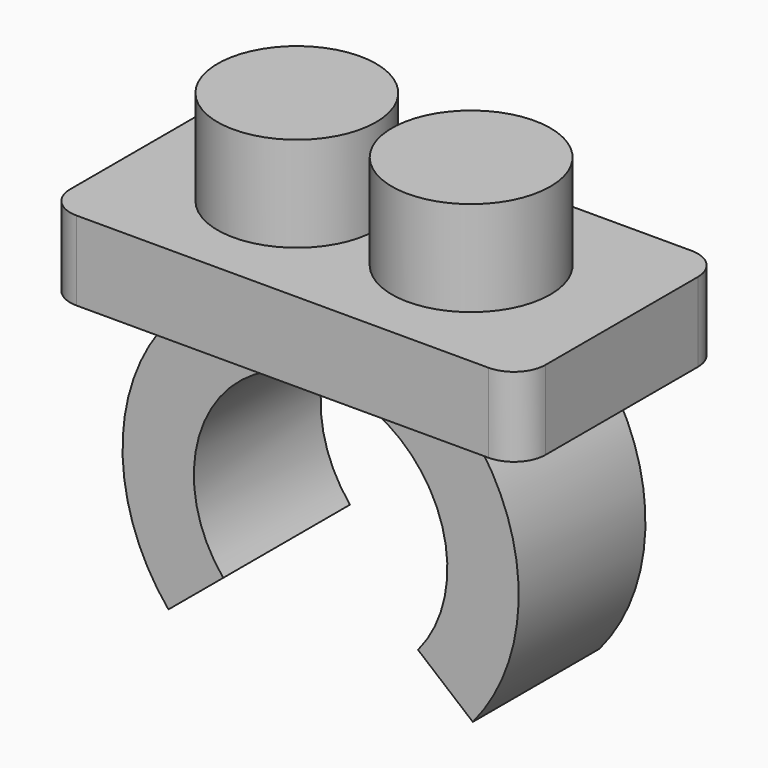
from build123d import *

# Parameters (mm, degrees)
F0_R     = 2.5
F1_DEPTH = 3
F2_W     = 15
F2_H     = 8
F3_DEPTH = 2.5
F5_DEPTH = 2.5
F6_R     = 1


with BuildPart() as f1:
    # F0 (on Top) → F1 (new body, symmetric)
    with BuildSketch(Plane.XY):
        with Locations((-2.75, 0)):
            Circle(F0_R)
    extrude(amount=F1_DEPTH, both=True)


with BuildPart() as f1b:
    # F0 (on Top) → F1, piece 2 (new body, symmetric)
    with BuildSketch(Plane.XY):
        with Locations((2.75, 0)):
            Circle(F0_R)
    extrude(amount=F1_DEPTH, both=True)


with BuildPart() as f3:
    # F2 (on Top) → F3 (new body)
    with BuildSketch(Plane.XY):
        Rectangle(F2_W, F2_H)
    extrude(amount=-F3_DEPTH)

    # F4 (on Front) → F5 (join, symmetric)
    with BuildSketch(Plane.XZ):
        with BuildLine():
            ThreePointArc((-3.073499634, -9.56), (0, -3), (3.073499634, -9.56))
            Line((3.073499634, -9.56), (4.8023431781, -11))
            ThreePointArc((4.8023431781, -11), (0, -0.75), (-4.8023431781, -11))
            Line((-4.8023431781, -11), (-3.073499634, -9.56))
        make_face()
    extrude(amount=F5_DEPTH, both=True)

    # F6
    f6_edges = [f3.edges().sort_by_distance(p)[0] for p in [
        (7.5, -4, -1.25),
        (-7.5, -4, -1.25),
        (7.5, 4, -1.25),
        (-7.5, 4, -1.25),
    ]]
    fillet(f6_edges, radius=F6_R)


solid = Compound([f1.part, f1b.part, f3.part])
